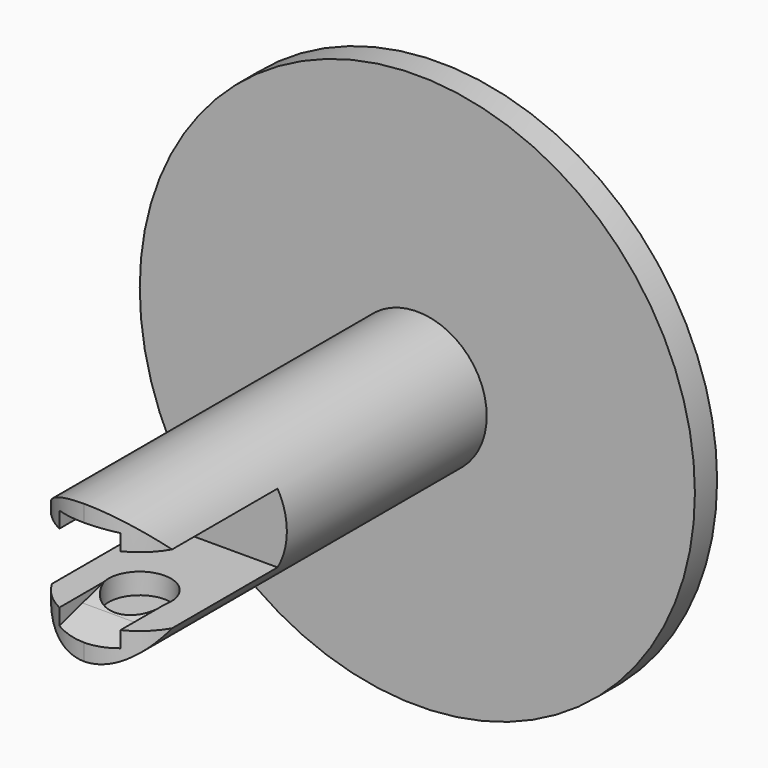
from build123d import *

# Parameters (mm, degrees)
F0_R           = 20
F1_DEPTH       = 2
F2_R           = 5
F3_DEPTH       = 30
F6_DEPTH       = 12
F7_R           = 2.25
F8_DEPTH       = 1.5
F8_DEPTH_BACK  = 6.5
F10_DEPTH      = 17.501
F10_DEPTH_BACK = 22.501
F12_DEPTH      = 2.2
F12_DEPTH_BACK = 2.2
F15_R          = 3
F16_DEPTH      = 15


# Not quite as in the source:
# - a pattern or mirror of a feature is missing from the dataset's text; its kind, count and spacing are read off the source's solid


with BuildPart() as f1:
    # F0 (on Front) → F1 (new body)
    with BuildSketch(Plane.XZ):
        Circle(F0_R)
    extrude(amount=F1_DEPTH)

    # F2 (on face) → F3 (join)
    with BuildSketch(Plane.XZ.offset(2)):
        Circle(F2_R)
    extrude(amount=F3_DEPTH)

    # F5 (on face) → F6 (cut)
    with BuildSketch(Plane.XZ.offset(32)):
        with BuildLine():
            Line((4.3301270189, 2.5), (-4.3301270189, 2.5))
            ThreePointArc((-4.3301270189, 2.5), (-4.8296291314, 1.2940952255), (-5, 0))
            ThreePointArc((-5, 0), (-4.8296291314, -1.2940952255), (-4.3301270189, -2.5))
            Line((-4.3301270189, -2.5), (4.3301270189, -2.5))
            ThreePointArc((4.3301270189, -2.5), (4.8296291314, -1.2940952255), (5, 0))
            ThreePointArc((5, 0), (4.8296291314, 1.2940952255), (4.3301270189, 2.5))
        make_face()
    extrude(amount=-F6_DEPTH, mode=Mode.SUBTRACT)

    # F7 (on face) → F8 (cut, two sides)
    with BuildSketch(Plane(origin=(0, 0, 2.5), x_dir=(1, 0, 0), z_dir=(0, 0, -1))) as f8_sk:
        with Locations((0, 27)):
            Circle(F7_R)
    extrude(amount=-F8_DEPTH, mode=Mode.SUBTRACT)
    extrude(f8_sk.sketch, amount=F8_DEPTH_BACK, mode=Mode.SUBTRACT)

    # F9 (on face) → F10 (cut, two sides)
    with BuildSketch(Plane.XY.offset(-2.5)) as f10_sk:
        with BuildLine():
            Line((4.3301270189, -32), (4.3301270189, -29.5))
            ThreePointArc((4.3301270189, -29.5), (2.5, -31.3301270189), (0, -32))
            Line((0, -32), (4.3301270189, -32))
        make_face()
        with BuildLine():
            Line((-4.3301270189, -32), (0, -32))
            ThreePointArc((0, -32), (-2.5, -31.3301270189), (-4.3301270189, -29.5))
            Line((-4.3301270189, -29.5), (-4.3301270189, -32))
        make_face()
    extrude(amount=-F10_DEPTH, mode=Mode.SUBTRACT)
    extrude(f10_sk.sketch, amount=F10_DEPTH_BACK, mode=Mode.SUBTRACT)

    # F11 (on Right) → F12 (cut, two sides)
    with BuildSketch(Plane.YZ) as f12_sk:
        Polygon((-32, 2.5), (-29.5, 2.5), (-29.4072434941, 3.0565390355), (-32, 3.8), align=None)
        Polygon((-29.5, 2.5), (-27.466361223, 2.5), (-29.4072434941, 3.0565390355), align=None)
    f12 = extrude(amount=-F12_DEPTH, mode=Mode.SUBTRACT) + extrude(f12_sk.sketch, amount=F12_DEPTH_BACK, mode=Mode.SUBTRACT)

    # F12_copies: F12 across plane
    add(f12.mirror(Plane(origin=(0, 0, 0), x_dir=(-1, 0, 0), z_dir=(0, 0, -1))), mode=Mode.SUBTRACT)

    # F15 (on offset) → F16 (cut, through all)
    with BuildSketch(Plane.XZ.offset(17)):
        Circle(F15_R)
    extrude(amount=-F16_DEPTH, mode=Mode.SUBTRACT)


solid = f1.part
